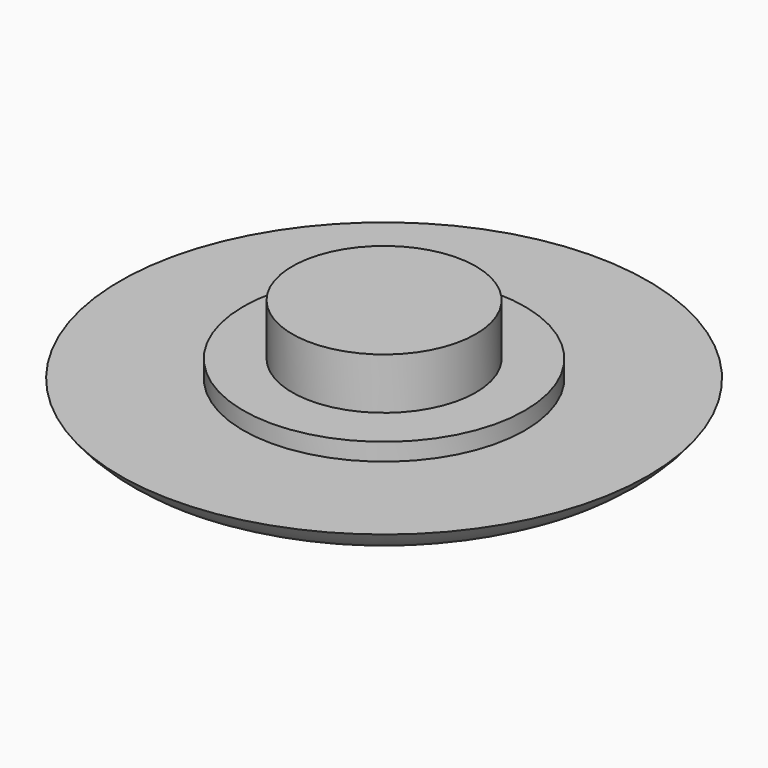
from build123d import *

# Parameters (mm, degrees)
F0_R     = 11.5
F1_DEPTH = 1.5
F3_R     = 6.1353913868
F3_R_2   = 4
F4_DEPTH = 0.762
F2_R     = 4
F5_DEPTH = 3


# Not quite as in the source:
# - a fillet or chamfer that OpenCascade refuses, or shapes differently, is made with other operations: its cross-section is extruded or revolved along the edge and cut away or added


with BuildPart() as f1:
    # F0 (on Top) → F1 (new body)
    with BuildSketch(Plane.XY):
        Circle(F0_R)
    extrude(amount=F1_DEPTH)

    # F3 (on face) → F4 (join)
    with BuildSketch(Plane.XY.offset(1.5)):
        Circle(F3_R)
        Circle(F3_R_2, mode=Mode.SUBTRACT)
    extrude(amount=F4_DEPTH)

    # F2 (on face) → F5 (join)
    with BuildSketch(Plane.XY.offset(1.5)):
        Circle(F2_R)
    extrude(amount=F5_DEPTH)

    # F6: fillet of radius 3.6792614691 on 1 edges, made by hand

    # F6_s1 → F6_t2 (revolve, cut)
    with BuildSketch(Plane.XZ):
        with BuildLine():
            ThreePointArc((11.5, 1.5), (10.1967383184, 0.396348303), (8.5355802579, 0))
            Line((8.5355802579, 0), (11.5, 0))
            Line((11.5, 0), (11.5, 1.5))
        make_face()
    revolve(axis=Axis((0, 0, 0), (0, 0, 1)), mode=Mode.SUBTRACT)


solid = f1.part
